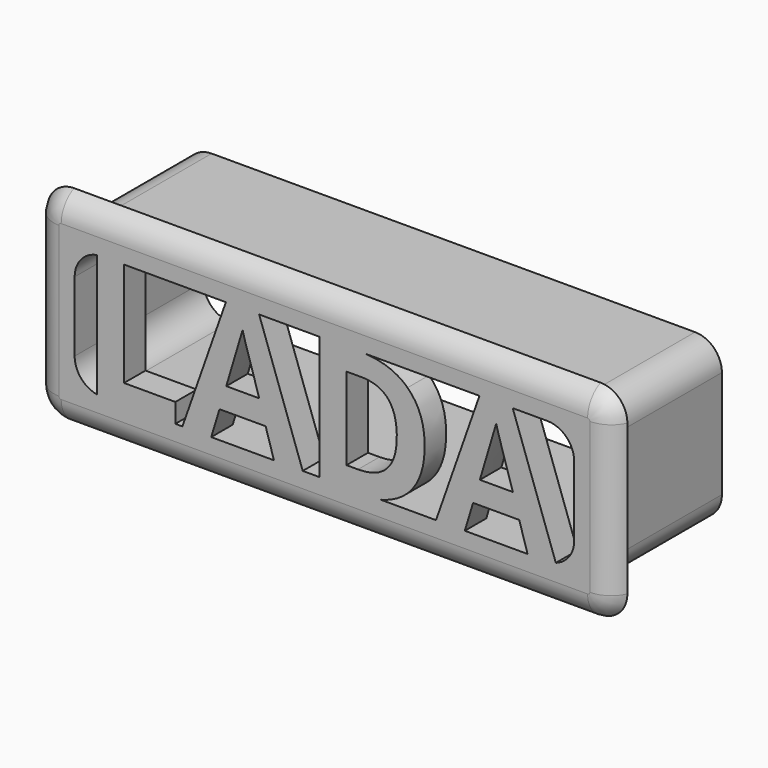
from build123d import *

# Parameters (mm, degrees)
F0_W         = 100
F0_H         = 30
F0_W_2       = 93
F0_H_2       = 23
F1_DEPTH     = 30
F2_W         = 100
F2_H         = 30
F3_DEPTH     = 3
F4_T1_DEPTH  = 28
F4_T3_DEPTH  = 98
F4_T6_ANGLE  = 90
F4_T8_ANGLE  = 90
F4_T10_ANGLE = 90
F4_T12_ANGLE = 90
F5_R         = 5
F7_DEPTH     = 25
F8_T         = -4
F11_DEPTH    = 5


# Not quite as in the source:
# - a fillet or chamfer that OpenCascade refuses, or shapes differently, is made with other operations: its cross-section is extruded or revolved along the edge and cut away or added
# - the program builds the solid bodies; features that only make, move or delete a surface that nothing else refers to are left out


with BuildPart() as f1:
    # F0 (on Front) → F1 (new body)
    with BuildSketch(Plane.XZ):
        with Locations((50, 15)):
            Rectangle(F0_W, F0_H)
        with Locations((50, 15)):
            Rectangle(F0_W_2, F0_H_2, mode=Mode.SUBTRACT)
    extrude(amount=F1_DEPTH)

    # F2 (on face) → F3 (join)
    with BuildSketch(Plane.XZ.offset(30)):
        with BuildLine():
            Line((99, 34), (1, 34))
            ThreePointArc((1, 34), (-2.5355339059, 32.5355339059), (-4, 29))
            Line((-4, 29), (-4, 1))
            ThreePointArc((-4, 1), (-2.5355339059, -2.5355339059), (1, -4))
            Line((1, -4), (99, -4))
            ThreePointArc((99, -4), (102.5355339059, -2.5355339059), (104, 1))
            Line((104, 1), (104, 29))
            ThreePointArc((104, 29), (102.5355339059, 32.5355339059), (99, 34))
        make_face()
        with Locations((50, 15)):
            Rectangle(F2_W, F2_H, mode=Mode.SUBTRACT)
    extrude(amount=-F3_DEPTH)

    # F4: fillet of radius 5 on 1 edges, made by hand

    # F4_s2 → F4_t1 (cut)
    with BuildSketch(Plane.XY.offset(1)):
        with BuildLine():
            ThreePointArc((104, -27), (102.1560370926, -29.1833001327), (99.417424305, -30))
            Line((99.417424305, -30), (104, -30))
            Line((104, -30), (104, -27))
        make_face()
        with BuildLine():
            ThreePointArc((-4, -27), (-2.1560370926, -29.1833001327), (0.582575695, -30))
            Line((0.582575695, -30), (-4, -30))
            Line((-4, -30), (-4, -27))
        make_face()
    extrude(amount=F4_T1_DEPTH, mode=Mode.SUBTRACT)

    # F4_s4 → F4_t3 (cut)
    with BuildSketch(Plane.YZ.offset(1)):
        with BuildLine():
            ThreePointArc((-27, 34), (-29.1833001327, 32.1560370926), (-30, 29.417424305))
            Line((-30, 29.417424305), (-30, 34))
            Line((-30, 34), (-27, 34))
        make_face()
        with BuildLine():
            ThreePointArc((-27, -4), (-29.1833001327, -2.1560370926), (-30, 0.582575695))
            Line((-30, 0.582575695), (-30, -4))
            Line((-30, -4), (-27, -4))
        make_face()
    extrude(amount=F4_T3_DEPTH, mode=Mode.SUBTRACT)

    # F4_s5 → F4_t6 (revolve, cut)
    with BuildSketch(Plane.XY.offset(29)):
        with BuildLine():
            ThreePointArc((104, -27), (102.1560370926, -29.1833001327), (99.417424305, -30))
            Line((99.417424305, -30), (104, -30))
            Line((104, -30), (104, -27))
        make_face()
    revolve(axis=Axis((99, -30, 29), (0, -1, 0)), revolution_arc=F4_T6_ANGLE, mode=Mode.SUBTRACT)

    # F4_s7 → F4_t8 (revolve, cut)
    with BuildSketch(Plane.YZ.offset(1)):
        with BuildLine():
            ThreePointArc((-27, 34), (-29.1833001327, 32.1560370926), (-30, 29.417424305))
            Line((-30, 29.417424305), (-30, 34))
            Line((-30, 34), (-27, 34))
        make_face()
    revolve(axis=Axis((1, -30, 29), (0, -1, 0)), revolution_arc=F4_T8_ANGLE, mode=Mode.SUBTRACT)

    # F4_s9 → F4_t10 (revolve, cut)
    with BuildSketch(Plane.XY.offset(1)):
        with BuildLine():
            ThreePointArc((-4, -27), (-2.1560370926, -29.1833001327), (0.582575695, -30))
            Line((0.582575695, -30), (-4, -30))
            Line((-4, -30), (-4, -27))
        make_face()
    revolve(axis=Axis((1, -30, 1), (0, -1, 0)), revolution_arc=F4_T10_ANGLE, mode=Mode.SUBTRACT)

    # F4_s11 → F4_t12 (revolve, cut)
    with BuildSketch(Plane.YZ.offset(99)):
        with BuildLine():
            ThreePointArc((-27, -4), (-29.1833001327, -2.1560370926), (-30, 0.582575695))
            Line((-30, 0.582575695), (-30, -4))
            Line((-30, -4), (-27, -4))
        make_face()
    revolve(axis=Axis((99, -30, 1), (0, -1, 0)), revolution_arc=F4_T12_ANGLE, mode=Mode.SUBTRACT)

    # F5
    f5_edges = [f1.edges().sort_by_distance(p)[0] for p in [
        (96.5, -15, 26.5),
        (96.5, -15, 3.5),
        (3.5, -15, 26.5),
        (3.5, -15, 3.5),
        (100, -13.5, 30),
        (0, -13.5, 30),
        (0, -13.5, 0),
        (100, -13.5, 0),
    ]]
    fillet(f5_edges, radius=F5_R)

    # F10 (on face) → F11 (join)
    with BuildSketch(Plane.XZ.offset(30)):
        with BuildLine():
            Line((7.6923411562, 26.5285422666), (7.6923411562, 26.4343375636))
            ThreePointArc((7.6923411562, 26.4343375636), (8.0948381917, 26.4835573549), (8.5, 26.5))
            Line((8.5, 26.5), (12.6897240143, 26.5))
            Line((12.6897240143, 26.5), (12.6897240143, 26.5285422666))
            Line((12.6897240143, 26.5285422666), (7.6923411562, 26.5285422666))
        make_face()
        Polygon((45.961234712, 3.5), (40.6030832841, 3.5), (40.7658357581, 2.9650311428), (46.1500129552, 2.9650311428), align=None)
        Polygon((31.649735074, 26.5), (23.5636409154, 3.5), (28.9224919537, 3.5), (30.4667918286, 8.5761276853), (39.0587834093, 8.5761276853), (40.6030832841, 3.5), (45.961234712, 3.5), (37.8450620877, 26.5), align=None)
        with BuildLine():
            add(Edge.make_bspline(
                [(37.8622995877, 12.7638210608), (35.4951182339, 20.3862481654), (35.1959972785, 21.3867561886)],
                knots=[0, 0, 0, 1, 1, 1], degree=2))
            Line((37.8622995877, 12.7638210608), (31.7251627444, 12.7638210608))
            add(Edge.make_bspline(
                [(34.7679448768, 22.9648770911), (34.2367473181, 20.9019739505), (31.7251627444, 12.7638210608)],
                knots=[0, 0, 0, 1, 1, 1], degree=2))
            add(Edge.make_bspline(
                [(35.1959972785, 21.3867561886), (34.8968763231, 22.3872642118), (34.7679448768, 22.9648770911)],
                knots=[0, 0, 0, 1, 1, 1], degree=2))
        make_face(mode=Mode.SUBTRACT)
        with BuildLine():
            Line((57.6041635325, 26.5), (49.1154362198, 26.5))
            Line((49.1154362198, 26.5), (49.1154362198, 3.5))
            Line((49.1154362198, 3.5), (60.4790861077, 3.5))
            add(Edge.make_bspline(
                [(65.3530625654, 6.0593858538), (63.4172768077, 4.2516481812), (60.4790861077, 3.5)],
                knots=[0, 0, 0, 0.5842050577, 0.5842050577, 0.5842050577], degree=2))
            add(Edge.make_bspline(
                [(68.666600735, 14.9711274212), (68.666600735, 9.1537405647), (65.3530625654, 6.0593858538)],
                knots=[0, 0, 0, 1, 1, 1], degree=2))
            add(Edge.make_bspline(
                [(65.4742581249, 23.4831815052), (68.666600735, 20.4378207439), (68.666600735, 14.9711274212)],
                knots=[0, 0, 0, 1, 1, 1], degree=2))
            add(Edge.make_bspline(
                [(57.6041635325, 26.5), (62.5909695012, 26.2337177448), (65.4742581249, 23.4831815052)],
                knots=[0.0968110332, 0.0968110332, 0.0968110332, 1, 1, 1], degree=2))
        make_face()
        with BuildLine():
            add(Edge.make_bspline(
                [(63.4732420785, 14.842195975), (63.4732420785, 22.4336795324), (56.7688068715, 22.4336795324)],
                knots=[0, 0, 0, 1, 1, 1], degree=2))
            add(Edge.make_bspline(
                [(56.2530810863, 7.0908374241), (63.4732420785, 7.0908374241), (63.4732420785, 14.842195975)],
                knots=[0, 0, 0, 1, 1, 1], degree=2))
            Line((56.2530810863, 7.0908374241), (54.1128190779, 7.0908374241))
            Line((54.1128190779, 7.0908374241), (54.1128190779, 22.4336795324))
            Line((54.1128190779, 22.4336795324), (56.7688068715, 22.4336795324))
        make_face(mode=Mode.SUBTRACT)
        with BuildLine():
            Line((93.3595513282, 2.9650311428), (93.0803262059, 3.7563127124))
            ThreePointArc((93.0803262059, 3.7563127124), (92.3004884639, 3.5644941273), (91.5, 3.5))
            Line((91.5, 3.5), (87.8126216572, 3.5))
            Line((87.8126216572, 3.5), (87.9753741312, 2.9650311428))
            Line((87.9753741312, 2.9650311428), (93.3595513282, 2.9650311428))
        make_face()
        with BuildLine():
            Line((85.0546004608, 26.5), (78.8592734471, 26.5))
            Line((78.8592734471, 26.5), (70.7731792884, 3.5))
            Line((70.7731792884, 3.5), (76.1320303268, 3.5))
            Line((76.1320303268, 3.5), (77.6763302017, 8.5761276853))
            Line((77.6763302017, 8.5761276853), (86.2683217823, 8.5761276853))
            Line((86.2683217823, 8.5761276853), (87.8126216572, 3.5))
            Line((87.8126216572, 3.5), (91.5, 3.5))
            ThreePointArc((91.5, 3.5), (92.3004884639, 3.5644941273), (93.0803262059, 3.7563127124))
            Line((93.0803262059, 3.7563127124), (85.0546004608, 26.5))
        make_face()
        with BuildLine():
            add(Edge.make_bspline(
                [(85.0718379608, 12.7638210608), (82.7046566069, 20.3862481654), (82.4055356515, 21.3867561886)],
                knots=[0, 0, 0, 1, 1, 1], degree=2))
            Line((85.0718379608, 12.7638210608), (78.9347011174, 12.7638210608))
            add(Edge.make_bspline(
                [(81.9774832498, 22.9648770911), (81.4462856911, 20.9019739505), (78.9347011174, 12.7638210608)],
                knots=[0, 0, 0, 1, 1, 1], degree=2))
            add(Edge.make_bspline(
                [(82.4055356515, 21.3867561886), (82.1064146961, 22.3872642118), (81.9774832498, 22.9648770911)],
                knots=[0, 0, 0, 1, 1, 1], degree=2))
        make_face(mode=Mode.SUBTRACT)
        with BuildLine():
            Line((7.6923411562, 26.4343375636), (7.6923411562, 3.5656624364))
            ThreePointArc((7.6923411562, 3.5656624364), (8.0948381917, 3.5164426451), (8.5, 3.5))
            Line((8.5, 3.5), (22.2461228132, 3.5))
            Line((22.2461228132, 3.5), (22.2461228132, 7.0908374241))
            Line((22.2461228132, 7.0908374241), (12.6897240143, 7.0908374241))
            Line((12.6897240143, 7.0908374241), (12.6897240143, 26.5))
            Line((12.6897240143, 26.5), (8.5, 26.5))
            ThreePointArc((8.5, 26.5), (8.0948381917, 26.4835573549), (7.6923411562, 26.4343375636))
        make_face()
    extrude(amount=-F11_DEPTH)


with BuildPart() as f7:
    # F6 (on Front) → F7 (new body)
    with BuildSketch(Plane.XZ):
        with BuildLine():
            add(Edge.make_bspline(
                [(-64.6141692996, 66.2774592638), (-57.3632405413, 65.4820326957), (-47.9649979836, 57.4179015801), (-35.44136599, 46.6694720335), (-22.7593679958, 45.2438805274), (-12.5503852984, 34.717586563), (-17.5949754851, 20.0575363254), (-41.16593926, 26.5737663135), (-51.8938502431, 42.0416927734), (-69.1953728198, 34.6634255071), (-93.0939149449, 45.9245842151), (-91.9481797024, 61.1508032719), (-73.0416739767, 67.2019561588), (-64.6141692996, 66.2774592638)],
                knots=[0, 0, 0, 0, 0.098374264, 0.187884813, 0.2668345062, 0.3470994933, 0.4198681033, 0.5217972145, 0.614123746, 0.7049715118, 0.8132456976, 0.8856629823, 1, 1, 1, 1], degree=3))
        make_face()
    extrude(amount=F7_DEPTH)

    # F8
    f8_openings = [f7.faces().sort_by_distance(p)[0] for p in [
        (-54.148596, -25, 45.943669),
    ]]
    offset(amount=F8_T, openings=f8_openings)


solid = f1.part
